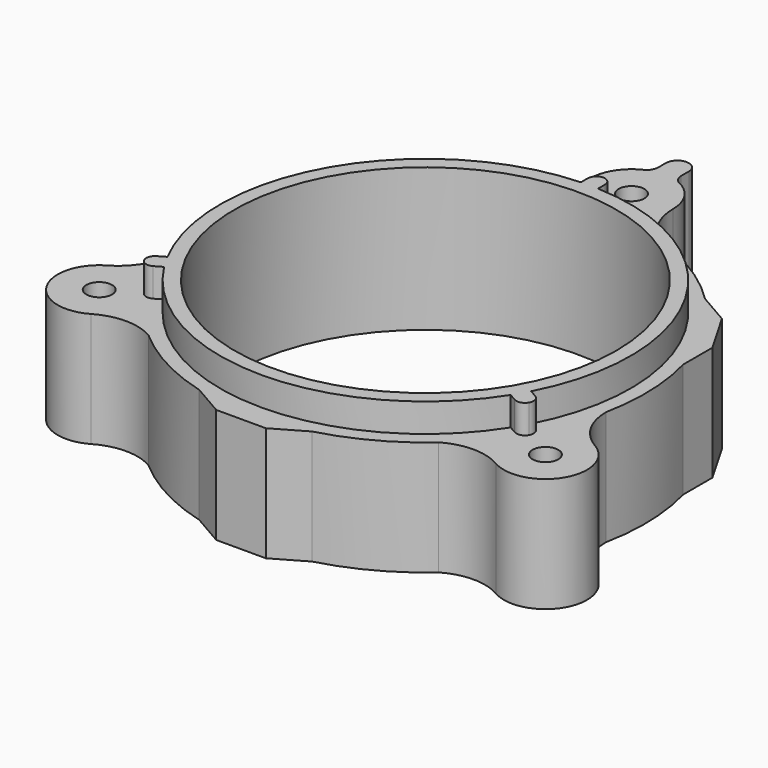
from build123d import *

# Parameters (mm, degrees)
F0_R     = 2.25
F0_R_2   = 33.35
F1_DEPTH = 20
F2_R     = 33.35
F3_DEPTH = 25
F5_DEPTH = 5
F6_R     = 1.49999
F7_SIZE  = 5
F8_R     = 1.99999


# Not quite as in the source:
# - a fillet or chamfer is up to 0.001 mm smaller than in the source, because OpenCascade refuses the exact size


with BuildPart() as f1:
    # F0 (on Top) → F1 (new body)
    with BuildSketch(Plane.XY):
        with BuildLine():
            ThreePointArc((-35.3461431703, -28.7786841774), (-30.3488782685, -27.4389385893), (-25.3508812473, -28.775950375))
            ThreePointArc((-25.3508812473, -28.775950375), (0, -38.35), (25.3508812473, -28.775950375))
            ThreePointArc((25.3508812473, -28.775950375), (30.3488782685, -27.4389385893), (35.3461431703, -28.7786841774))
            ThreePointArc((35.3461431703, -28.7786841774), (45.2498273477, -26.125), (42.5961431703, -16.2213158226))
            ThreePointArc((42.5961431703, -16.2213158226), (38.9372570055, -12.5634302623), (37.5961446665, -7.566531981))
            ThreePointArc((37.5961446665, -7.566531981), (33.2120742351, 19.175), (12.2452634191, 36.342482356))
            ThreePointArc((12.2452634191, 36.342482356), (8.588378737, 40.0023688516), (7.25, 45))
            ThreePointArc((7.25, 45), (5.790617411, 49.3624820917), (2, 51.9686799324))
            Line((2, 51.9686799324), (2, 54.1277186767))
            Line((2, 54.1277186767), (2, 57))
            Line((2, 57), (0, 57))
            Line((0, 57), (-2, 57))
            Line((-2, 57), (-2, 54.1277186767))
            Line((-2, 54.1277186767), (-2, 51.9686799324))
            ThreePointArc((-2, 51.9686799324), (-5.790617411, 49.3624820917), (-7.25, 45))
            ThreePointArc((-7.25, 45), (-8.588378737, 40.0023688516), (-12.2452634191, 36.342482356))
            ThreePointArc((-12.2452634191, 36.342482356), (-33.2120742351, 19.175), (-37.5961446665, -7.566531981))
            ThreePointArc((-37.5961446665, -7.566531981), (-38.9372570055, -12.5634302623), (-42.5961431703, -16.2213158226))
            ThreePointArc((-42.5961431703, -16.2213158226), (-45.2498273477, -26.125), (-35.3461431703, -28.7786841774))
        make_face()
        with Locations((-38.9711431703, -22.5)):
            Circle(F0_R, mode=Mode.SUBTRACT)
        with Locations((38.9711431703, -22.5)):
            Circle(F0_R, mode=Mode.SUBTRACT)
        Circle(F0_R_2, mode=Mode.SUBTRACT)
        with Locations((0, 45)):
            Circle(F0_R, mode=Mode.SUBTRACT)
    extrude(amount=F1_DEPTH)

    # F2 (on Top) → F3 (join)
    with BuildSketch(Plane.XY):
        Polygon((37.0225860118, -21.375), (37.0225860118, 21.375), (0, 42.75), (-37.0225860118, 21.375), (-37.0225860118, -21.375), (0, -42.75), align=None)
        Circle(F2_R, mode=Mode.SUBTRACT)
    extrude(amount=F3_DEPTH)

    # F4 (on face) → F5 (cut)
    with BuildSketch(Plane.XY.offset(25)):
        Polygon((37.0225860118, -21.375), (37.0225860118, 21.375), (0, 42.75), (-37.0225860118, 21.375), (-37.0225860118, -21.375), (0, -42.75), align=None)
        with BuildLine():
            ThreePointArc((-31.7698222916, -16.6102646446), (-31.0470107257, 17.925), (-1.5, 35.8186055005))
            Line((-1.5, 35.8186055005), (-1.5, 38.8186055005))
            Line((-1.5, 38.8186055005), (0, 38.8186055005))
            Line((0, 38.8186055005), (1.5, 38.8186055005))
            Line((1.5, 38.8186055005), (1.5, 35.8186055005))
            ThreePointArc((1.5, 35.8186055005), (31.0470107257, 17.925), (31.7698222916, -16.6102646446))
            Line((31.7698222916, -16.6102646446), (34.3678985029, -18.1102646446))
            Line((34.3678985029, -18.1102646446), (33.6178985029, -19.4093027502))
            Line((33.6178985029, -19.4093027502), (32.8678985029, -20.7083408559))
            Line((32.8678985029, -20.7083408559), (30.2698222916, -19.2083408559))
            ThreePointArc((30.2698222916, -19.2083408559), (0, -35.85), (-30.2698222916, -19.2083408559))
            Line((-30.2698222916, -19.2083408559), (-32.8678985029, -20.7083408559))
            Line((-32.8678985029, -20.7083408559), (-33.6178985029, -19.4093027502))
            Line((-33.6178985029, -19.4093027502), (-34.3678985029, -18.1102646446))
            Line((-34.3678985029, -18.1102646446), (-31.7698222916, -16.6102646446))
        make_face(mode=Mode.SUBTRACT)
    extrude(amount=-F5_DEPTH, mode=Mode.SUBTRACT)

    # F6 (radius 1.5 in the source; OpenCascade refuses exactly that, so slightly less here)
    f6_edges = [f1.edges().sort_by_distance(p)[0] for p in [
        (-32.867899, -20.708341, 22.5),
        (-34.367899, -18.110265, 22.5),
        (32.867899, -20.708341, 22.5),
        (34.367899, -18.110265, 22.5),
        (1.5, 38.818606, 22.5),
        (-1.5, 38.818606, 22.5),
    ]]
    fillet(f6_edges, radius=F6_R)

    # F7
    f7_edges = [f1.edges().sort_by_distance(p)[0] for p in [
        (0, -42.75, 10),
        (37.022586, 21.375, 10),
        (-37.022586, 21.375, 10),
    ]]
    chamfer(f7_edges, length=F7_SIZE)

    # F8 (radius 2 in the source; OpenCascade refuses exactly that, so slightly less here)
    f8_edges = [f1.edges().sort_by_distance(p)[0] for p in [
        (-2, 57, 10),
        (2, 57, 10),
        (-2, 51.96868, 10),
        (2, 51.96868, 10),
    ]]
    fillet(f8_edges, radius=F8_R)


solid = f1.part
